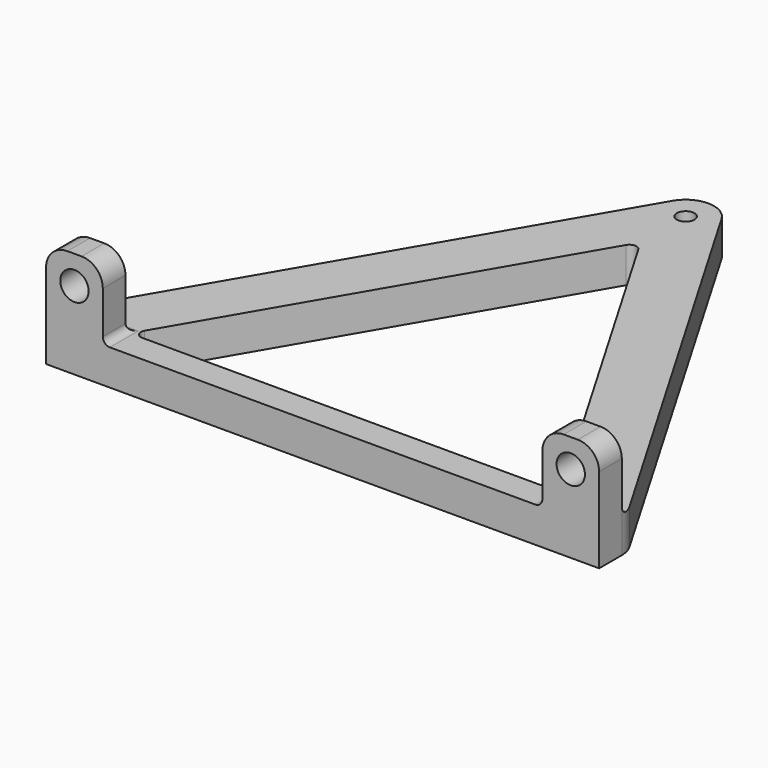
from build123d import *

# Parameters (mm, degrees)
F0_R     = 1.25
F1_DEPTH = 5
F2_R     = 2
F3_DEPTH = 4
F5_R     = 1


with BuildPart() as f1:
    # F0 (on Top) → F1 (new body)
    with BuildSketch(Plane.XY):
        with BuildLine():
            ThreePointArc((3.4551156036, 66.0154841021), (0, 68), (-3.4551156036, 66.0154841021))
            Line((-3.4551156036, 66.0154841021), (-38.4551156036, 6.0154841021))
            ThreePointArc((-38.4551156036, 6.0154841021), (-38.8613768538, 5.0439199169), (-39, 4))
            Line((-39, 4), (-39, 0))
            Line((-39, 0), (39, 0))
            Line((39, 0), (39, 4))
            ThreePointArc((39, 4), (38.8613768538, 5.0439199169), (38.4551156036, 6.0154841021))
            Line((38.4551156036, 6.0154841021), (3.4551156036, 66.0154841021))
        make_face()
        with BuildLine():
            Line((-29.4919272386, 5.5038710255), (-0.8637789009, 54.5806967473))
            ThreePointArc((-0.8637789009, 54.5806967473), (0, 55.0768257218), (0.8637789009, 54.5806967473))
            Line((0.8637789009, 54.5806967473), (29.4919272386, 5.5038710255))
            ThreePointArc((29.4919272386, 5.5038710255), (29.4952904903, 4.5019392735), (28.6281483377, 4))
            Line((28.6281483377, 4), (-28.6281483377, 4))
            ThreePointArc((-28.6281483377, 4), (-29.4952904903, 4.5019392735), (-29.4919272386, 5.5038710255))
        make_face(mode=Mode.SUBTRACT)
        with Locations((0, 64)):
            Circle(F0_R, mode=Mode.SUBTRACT)
    extrude(amount=F1_DEPTH)

    # F2 (on Front) → F3 (join)
    with BuildSketch(Plane.XZ):
        with BuildLine():
            Line((-39, 12), (-39, 0))
            Line((-39, 0), (-31, 0))
            Line((-31, 0), (-31, 12))
            ThreePointArc((-31, 12), (-31.8786796564, 14.1213203436), (-34, 15))
            Line((-34, 15), (-36, 15))
            ThreePointArc((-36, 15), (-38.1213203436, 14.1213203436), (-39, 12))
        make_face()
        with Locations((-35, 11)):
            Circle(F2_R, mode=Mode.SUBTRACT)
    extrude(amount=-F3_DEPTH)

    # F4: F1 across plane


with BuildPart() as f1_1:
    add(f1.part)
    add(f1.part.mirror(Plane.YZ))

    # F5
    f5_edges = [f1_1.edges().sort_by_distance(p)[0] for p in [
        (-35, 4, 5),
        (-31, 2, 5),
        (31, 2, 5),
        (35, 4, 5),
    ]]
    fillet(f5_edges, radius=F5_R)


solid = f1_1.part
